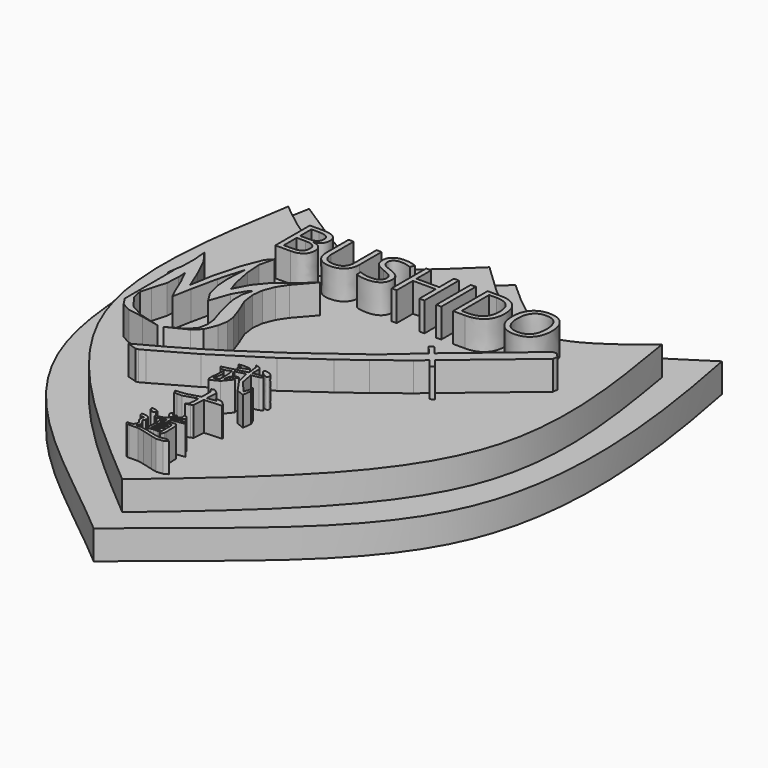
from build123d import *

# Parameters (mm, degrees)
F1_DEPTH     = 2.54
F3_DEPTH     = 5.08
F4_TEXT_SIZE = 5.2916666667
F8_DEPTH     = 2.54
F9_DEPTH     = 2.54
F10_DEPTH    = 2.54


# Not quite as in the source:
# - Text() gives the source's letters only with a copy of the font that has no kerning and outlines rounded to 1/6400 em; it was checked with that copy


with BuildPart() as f1:
    # F0 (on Top) → F1 (new body)
    with BuildSketch(Plane.XY):
        with BuildLine():
            add(Edge.make_bspline(
                [(0, 0), (3.7131397824, -3.5052822794), (8.5608695989, -5.628524388), (10.9297987074, -4.6822023578), (18.0759746581, 0)],
                knots=[0, 0, 0, 0, 0.4720166687, 1, 1, 1, 1], degree=3))
            add(Edge.make_bspline(
                [(0, 0), (-3.7131397824, -3.5052822794), (-8.5608695989, -5.628524388), (-10.9297987074, -4.6822023578), (-18.0759746581, 0)],
                knots=[0, 0, 0, 0, 0.4720166687, 1, 1, 1, 1], degree=3))
            add(Edge.make_bspline(
                [(-18.0759746581, 0), (-19.8166941403, -8.9087871241), (-22.9591659996, -30.0071749991), (-6.94082423, -40.2375085159), (0, -46.1805574596)],
                knots=[0, 0, 0, 0, 0.5071458871, 1, 1, 1, 1], degree=3))
            add(Edge.make_bspline(
                [(18.0759746581, 0), (19.8166941403, -8.9087871241), (22.9591659996, -30.0071749991), (6.94082423, -40.2375085159), (0, -46.1805574596)],
                knots=[0, 0, 0, 0, 0.5071458871, 1, 1, 1, 1], degree=3))
        make_face()
    extrude(amount=F1_DEPTH)

    # F2 (on Top) → F3 (join)
    with BuildSketch(Plane.XY):
        with BuildLine():
            add(Edge.make_bspline(
                [(0, -2.8561118525), (2.8233653699, -5.6129188632), (8.2844687451, -10.9452815222), (13.7327375569, -6.5557824481), (16.3642764091, -4.4356342405)],
                knots=[0, 0, 0, 0, 0.5169954084, 1, 1, 1, 1], degree=3))
            add(Edge.make_bspline(
                [(0, -2.8561118525), (-2.8233653699, -5.6129188632), (-8.2844687451, -10.9452815222), (-13.7327375569, -6.5557824481), (-16.3642764091, -4.4356342405)],
                knots=[0, 0, 0, 0, 0.5169954084, 1, 1, 1, 1], degree=3))
            add(Edge.make_bspline(
                [(-16.3642764091, -4.4356342405), (-17.5306592497, -11.405154188), (-19.9903582683, -26.1026623973), (-6.8888220266, -37.2177760295), (0, -43.0621318519)],
                knots=[0, 0, 0, 0, 0.4741973842, 1, 1, 1, 1], degree=3))
            add(Edge.make_bspline(
                [(16.3642764091, -4.4356342405), (17.5306592497, -11.405154188), (19.9903582683, -26.1026623973), (6.8888220266, -37.2177760295), (0, -43.0621318519)],
                knots=[0, 0, 0, 0, 0.4741973842, 1, 1, 1, 1], degree=3))
        make_face()
    extrude(amount=F3_DEPTH)

    # F4 (on face) + F7 (on face) → F8 (join)
    with BuildSketch(Plane.XY.offset(5.08)):
        with Locations((-10.92195604, -13.2894301787)):
            Text('BUSHIDO', F4_TEXT_SIZE, font='Open Sans', text_align=(TextAlign.LEFT, TextAlign.BOTTOM))
    with BuildSketch(Plane.XY.offset(5.08)):
        Polygon((8.0822174559, -18.9671691951), (7.4287134977, -18.1892682273), (7.135406261, -18.4356716232), (7.7889102193, -19.2135725911), (5.1391113657, -21.5436444753), (3.686977524, -22.614869239), (1.8583918329, -23.9637988065), (0.3626892216, -25.0671638204), (-1.4275072423, -26.278417952), (-2.9584097022, -27.3084261391), (-4.9349892273, -28.5482173422), (-6.7204780085, -29.5908928712), (-9.1772713105, -30.9231481988), (-8.3163375336, -31.1967801574), (-8.0879192873, -31.1420760859), (-7.6503931534, -30.911703117), (-4.3108317337, -29.0299077777), (0.0929313638, -26.2266536212), (3.2696862571, -23.9877574758), (5.234673525, -22.538205815), (7.6208872753, -20.6816272902), (8.4424142872, -19.9914736893), (9.0235599966, -20.6832427354), (9.3249463854, -20.4464563895), (8.7357215238, -19.7450702934), (14.9206722544, -14.5491778193), (14.9680923331, -14.1395488087), (14.6466968495, -13.7569744499), (14.2671681866, -13.771276721), align=None)
    extrude(amount=F8_DEPTH)

    # F7 (on face) → F9 (join)
    with BuildSketch(Plane.XY.offset(5.08)):
        Polygon((-9.4831661239, -16.2324859195), (-9.1647897509, -14.9246578416), (-9.6441104099, -15.4305585414), (-10.2958255982, -17.0849084154), (-10.9136704713, -19.3274537854), (-11.302683563, -21.489908032), (-11.9891770341, -19.8194407106), (-12.7443191032, -18.2290640444), (-13.533787344, -17.1421163607), (-13.4308125743, -18.3892462913), (-13.4536948161, -19.6478173428), (-13.6596424828, -20.9635968078), (-13.5331712332, -20.5185325796), (-13.5331712332, -25.8682832801), (-13.0761237815, -26.5585184097), (-12.2980975979, -26.9704137433), (-10.9251106558, -27.2106857091), (-9.3168115839, -27.5610884194), (-11.1706860432, -27.0570082062), (-12.3444688289, -26.4027697259), (-13.1815105594, -25.2770932066), (-13.3482236184, -24.4387655224), (-13.0852980267, -23.5164199644), (-12.719693399, -22.2464265188), (-12.6427244965, -21.0918873632), (-12.6965874409, -20.3172421644), (-12.1111528054, -21.4900025396), (-11.4689417108, -23.0257411042), (-11.1806855193, -23.6031846289), (-10.8724303756, -21.9385490361), (-10.3817515154, -19.6487124825), (-10.1027376053, -18.6288693745), (-9.7464252014, -17.4293836271), (-9.8540048842, -19.1804589308), (-9.7677047334, -20.4216090078), (-9.4499167416, -21.6434769196), (-8.8822671062, -22.5574875526), (-8.285755771, -20.8256778829), (-7.7181061356, -19.8539401049), (-7.3813650804, -19.4979572923), (-7.631515418, -20.3638625953), (-7.631515418, -21.402948397), (-7.4375607008, -22.3782625682), (-7.1312147427, -23.5099817005), (-6.8040955026, -24.5298257448), (-6.7271247274, -25.3091393939), (-6.87144259, -26.0788331006), (-7.3813650804, -26.6849671872), (-8.8447894305, -27.4931017839), (-7.1360846582, -26.6401270615), (-6.4789925104, -26.0369626245), (-6.0624479449, -24.9795828645), (-5.9022666343, -24.1443492038), (-6.0008237587, -23.3910273768), (-6.347186629, -22.400046905), (-6.8859708192, -21.0530836205), (-7.0302886818, -19.9947560613), (-6.9244562068, -19.0615027345), (-6.549229764, -18.1090071821), (-6.0008237587, -17.2719659198), (-4.6073853097, -15.6726494589), (-5.7121880335, -16.6754536483), (-7.0880158268, -17.7337816757), (-8.0693735472, -18.9268057507), (-8.7428556576, -20.2064210113), (-9.0507331403, -19.3020312571), (-9.3874741955, -17.6087065069), align=None)
    extrude(amount=F9_DEPTH)

    # F6 (on face) → F10 (join)
    with BuildSketch(Plane.XY.offset(5.08)):
        with BuildLine():
            add(Edge.make_bspline(
                [(-1.3619952315, -28.6367721492), (-1.3356277462, -28.5573903318), (0.5285441317, -28.5069084276), (-1.5223925511, -29.1696131573), (-0.6615029748, -28.8255790907), (-1.3799571802, -28.6908483005), (-1.3619952315, -28.6367721492)],
                knots=[0, 0, 0, 0, 0.323818666, 0.6224903435, 0.7794095959, 1, 1, 1, 1], degree=3))
        make_face()
        with BuildLine():
            add(Edge.make_bspline(
                [(0.6040885938, -28.3234266691), (0.5689610038, -28.4786050119), (1.4143065093, -29.1886421157), (1.4533251214, -28.3174201121), (0.6356142275, -28.1841601953), (0.6040885938, -28.3234266691)],
                knots=[0, 0, 0, 0, 0.3876451352, 0.6521037019, 1, 1, 1, 1], degree=3))
        make_face()
        Polygon((-0.0054208097, -28.0584224778), (-0.3234248936, -27.9877548797), (-0.1555896437, -28.2350920103), (-0.0584217769, -29.1007721822), (-1.7897821208, -29.5512791139), (-2.1431207559, -29.6307801349), (-1.9222845388, -29.8781172655), (-1.5689441843, -29.8781172655), (-1.0831048505, -29.6837811021), (-1.0036033997, -30.2314563305), (-1.0036033997, -31.1148033482), (-1.4629439692, -31.2914726657), (-1.3216074835, -30.4964603068), (-1.3834425184, -30.2402895384), (-1.5689441843, -30.0282865293), (-1.5689441843, -30.2844568678), (-1.6464593718, -31.1678038855), (-1.6464593718, -31.4940828767), (-1.5512777683, -31.6889786303), (-0.7915995308, -31.3179731493), (-0.1555896437, -30.5317944282), (-0.429426828, -30.761464713), (-0.7915995308, -30.9293003928), (-0.6944316641, -30.3992920102), (-0.2792579941, -30.3992920102), (-0.1114227441, -30.1166211881), (-0.3587594449, -30.1166211881), (-0.6767652481, -30.2137894847), (-0.6767652481, -30.0547870129), (-0.8533118278, -29.8802126969), (-0.9186822668, -29.6167491072), (-0.0495877093, -29.4011098501), (0.241915891, -30.5759617576), (1.0104281961, -31.6889786303), (1.6906049828, -31.9628166743), (1.7877745689, -31.1854711611), (1.5669366325, -30.6907969), (1.5669366325, -31.1324701939), (1.4167677985, -31.5388097963), (0.5051495483, -30.4889654245), (0.2949168582, -29.3569425207), (0.9132603294, -29.2421073783), (1.1870975137, -29.0919385444), (0.9662612966, -28.9241028646), (0.1977489914, -29.0566048528), (0.1977489914, -28.2615924939), align=None)
        Polygon((-0.3234248936, -32.583967859), (-0.5323889354, -32.6508208438), (-0.3234248936, -33.0073660839), (-0.3234248936, -33.9432984137), (-1.4088976316, -34.2701314071), (-2.3225444869, -34.3666957788), (-2.2010674511, -34.6130776129), (-1.9140023854, -34.648961262), (-1.4980326521, -34.648961262), (-0.3320604135, -34.2849875304), (-0.3320604135, -34.7696381644), (-0.3912570534, -35.2432044751), (-0.5992410604, -35.4586169735), (-0.1906989589, -35.3397688467), (-0.0049978474, -35.2283483518), (0.0692819095, -34.2107077736), (1.5920289609, -34.1141434019), (1.5920289609, -34.0027229069), (1.1672589792, -33.6200082413), (0.6041006293, -33.5496124355), (0.7682451943, -33.7442887327), (0.8566538659, -33.7798819169), (0.0618542777, -33.8913024119), (0.1287064027, -32.9033732207), (-0.1553355873, -32.6516403344), align=None)
        Polygon((-1.5481828491, -37.3994832672), (-1.9547941828, -37.3486561198), (-1.9106272833, -37.5518259209), (-1.625792851, -37.7113427367), (-1.7101817415, -37.7308708435), (-1.6986234145, -37.8300801391), (-1.3412347463, -37.6851064771), (-1.3894516789, -37.476741504), align=None)
        Polygon((-0.2952204019, -37.1481172204), (-0.3234248936, -37.0262341424), (-0.4707722591, -37.1145688012), (-0.4707722591, -37.2868210849), (-0.3647703247, -37.4944079199), (-0.1076088398, -37.6653383262), (0.0945702449, -37.1631527345), (-0.1571834897, -37.3221556362), align=None)
        Polygon((0.7141215134, -36.8989339109), (0.5030951528, -36.8725552366), (0.5088309351, -36.8651233064), (0.4776004943, -36.9026010389), (0.4991421677, -36.9963681258), (0.5338149439, -37.1462032914), (0.1246899796, -37.5834371998), (-0.3593921691, -37.9176092781), (-0.827857378, -38.0643961325), (-1.0870748509, -38.0643961325), (-1.0714579111, -38.1861963991), (-0.9652737246, -38.301751953), (-0.7841323538, -38.3204903894), (-0.0220951554, -38.0269184), (-0.39411811, -38.5358242751), (-0.3288626536, -38.722892339), (-0.3734272984, -39.0794043717), (-0.4168930167, -39.5811891265), (-0.301595909, -39.9117117812), (-0.1381605064, -39.8159564789), (0.1184624605, -39.7860587545), (0.4614727782, -39.7860587545), (0.6337733307, -39.7461873501), (0.6556349831, -39.6962176132), (0.5853664913, -39.5712924112), (0.4196407914, -39.5407533843), (0.1122160285, -39.6118933598), (-0.0736088769, -39.5900317073), (-0.062677191, -39.5603624447), (-0.1969711813, -39.6150157161), (-0.1805404768, -39.34022716), (-0.1472834193, -39.2576211126), (0.2705432219, -39.292904083), (0.1293353207, -39.4354356582), (0.1498373275, -39.4637482116), (0.3113969163, -39.3467578524), (0.5512934108, -39.2347264428), (0.5936623995, -39.1294875863), (0.5063825676, -39.0596781412), (0.3431415265, -39.0596781412), (0.0254176172, -39.1332014022), (-0.1695680341, -39.1350583102), (-0.1695680341, -38.9010750128), (0.0670709959, -38.9027468695), (0.1182681729, -38.9233587679), (0.030988341, -38.9976402442), (0.0625574956, -39.0199231396), (0.1873863914, -38.9333212835), (0.4395304425, -38.8453651951), (0.5416655381, -38.7432292399), (0.4599581494, -38.6633778995), (0.3336815311, -38.6540925001), (0.1184026891, -38.7033318213), (-0.1403941382, -38.7397032184), (-0.1547110511, -38.69866087), (-0.2029940967, -38.518531342), (-0.0785743863, -38.4368230936), (0.1149962324, -38.4368230936), (0.4153830964, -38.4761262261), (0.6388976317, -38.4244035919), (0.7137699569, -38.6390403698), (0.7137699569, -38.8780252831), (0.7137699569, -39.8313386153), (0.8777606009, -40.0272040653), (1.0081470784, -39.703341632), (1.0289147464, -39.537202676), (0.9901586703, -38.4056072674), (0.7839679037, -38.1804563496), (0.4107724403, -38.2329053712), (0.0857963548, -38.3276128349), (0.132220773, -38.2607607099), (0.1564310701, -37.9500252171), (1.3119797317, -37.787624002), (1.1511568502, -37.6289558705), (1.0134124712, -37.5735002124), (0.6498820072, -37.6158531388), (0.1580158889, -37.7874321213), (-0.0153397931, -37.7657623495), (0.3875404586, -37.587745914), (0.8708513295, -37.2124284353), (0.8435145228, -37.094294977), align=None)
        Polygon((-1.7737422186, -38.4267889133), (-1.9835367109, -38.4510808799), (-1.9828162993, -38.5149722684), (-1.9320229894, -38.6342244446), (-1.7973146335, -38.7601193652), (-1.6205077672, -38.7601193652), (-1.5154600771, -38.7758764327), (-1.5994971975, -38.9807208898), (-1.5522268546, -39.2643506845), (-1.3263718279, -39.5847481164), (-1.3263718279, -39.8106014238), (-1.4839442227, -40.0154458808), (-1.7203028148, -40.0574653007), (-1.9303999143, -40.031203808), (-1.9303999143, -40.1940271258), (-1.7885854467, -40.2938238928), (-1.636263975, -40.2938238928), (-0.8536546437, -40.2728133232), (-0.2391229919, -40.4041242253), (0.6170198945, -40.635230175), (1.137009141, -40.7560357923), (1.6885125227, -40.6877548797), (2.0351714472, -40.5039209923), (1.8303269902, -40.3515995206), (1.6149789677, -40.3515995206), (1.1265038562, -40.4356383604), (0.5907584018, -40.3305906703), (-0.1218816063, -40.1471075322), (-0.7910166681, -40.0300638729), (-1.2371078555, -40.0300638729), (-1.1023960609, -39.9218542812), (-1.0582291613, -39.7186844801), (-1.1090224713, -39.5155146789), (-1.3232357167, -39.1665913582), (-1.199565647, -38.9744641416), (-1.199565647, -38.7712943404), (-1.3011505476, -38.5924165059), (-1.5440719338, -38.4577064307), align=None)
    extrude(amount=F10_DEPTH)


solid = f1.part
